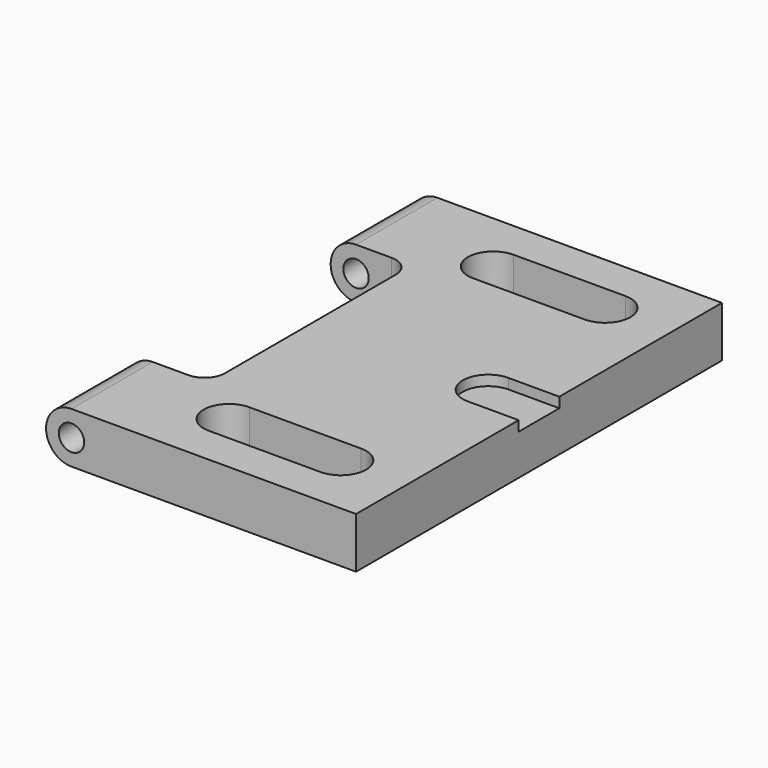
from build123d import *

# Parameters (mm, degrees)
F1_DEPTH = 5
F3_D     = 5
F4_R     = 4.99999
F5_R     = 4
F7_DEPTH = 2


# Not quite as in the source:
# - a fillet or chamfer is up to 0.001 mm smaller than in the source, because OpenCascade refuses the exact size
# - a feature names something its author has since deleted; it is built from what else it names


with BuildPart() as f1:
    # F0 (on Top) → F1 (new body, symmetric)
    with BuildSketch(Plane.XY):
        Polygon((13, -45), (56, -45), (56, 45), (13, 45), (-5, 45), (-5, 25), (11, 25), (11, -25), (-5, -25), (-5, -45), align=None)
        with BuildLine():
            ThreePointArc((43, -27.5), (48, -32.5), (43, -37.5))
            Line((43, -37.5), (21, -37.5))
            ThreePointArc((21, -37.5), (16, -32.5), (21, -27.5))
            Line((21, -27.5), (43, -27.5))
        make_face(mode=Mode.SUBTRACT)
        with BuildLine():
            ThreePointArc((43, 37.5), (48, 32.5), (43, 27.5))
            Line((43, 27.5), (21, 27.5))
            ThreePointArc((21, 27.5), (16, 32.5), (21, 37.5))
            Line((21, 37.5), (43, 37.5))
        make_face(mode=Mode.SUBTRACT)
    extrude(amount=F1_DEPTH, both=True)

    # F3 (through all)
    with Locations(Plane.XZ.offset(45)):
        with Locations((0, 0)):
            Hole(F3_D / 2)

    # F4 (radius 5 in the source; OpenCascade refuses exactly that, so slightly less here)
    f4_edges = [f1.edges().sort_by_distance(p)[0] for p in [
        (-5, -35, 5),
        (-5, -35, -5),
        (-5, 35, 5),
        (-5, 35, -5),
    ]]
    fillet(f4_edges, radius=F4_R)

    # F5
    f5_edges = [f1.edges().sort_by_distance(p)[0] for p in [
        (11, 25, 0),
        (11, -25, 0),
    ]]
    fillet(f5_edges, radius=F5_R)

    # F6 (on face) → F7 (cut)
    with BuildSketch(Plane.XY.offset(5)):
        with BuildLine():
            ThreePointArc((46, 5), (41, 0), (46, -5))
            Line((46, -5), (56, -5))
            Line((56, -5), (56, 5))
            Line((56, 5), (46, 5))
        make_face()
    extrude(amount=-F7_DEPTH, mode=Mode.SUBTRACT)


solid = f1.part
